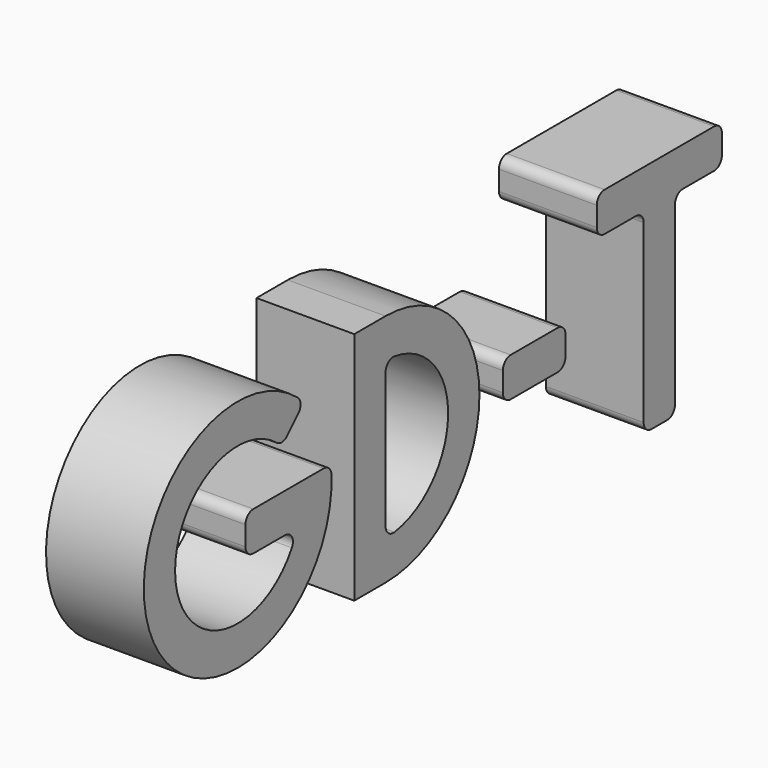
from build123d import *

# Parameters (mm, degrees)
F1_DEPTH = 10
F0_W     = 8
F0_H     = 4
F2_R     = 1
F3_R     = 1
F4_R     = 1
F4_2_R   = 1
F4_3_R   = 1


with BuildPart() as f1:
    # F0 (on Right) → F1 (new body)
    with BuildSketch(Plane.YZ):
        with BuildLine():
            Line((17.6568542495, 17.6568542495), (20.4852813742, 20.4852813742))
            ThreePointArc((20.4852813742, 20.4852813742), (1.2227826555, 6.7225397861), (23.9058808998, 13.5))
            Line((23.9058808998, 13.5), (13, 13.5))
            Line((13, 13.5), (13, 9.5))
            Line((13, 9.5), (19.5993420768, 9.5))
            ThreePointArc((19.5993420768, 9.5), (4.217631911, 10.1466929753), (17.6568542495, 17.6568542495))
        make_face()
    extrude(amount=F1_DEPTH)

    # F3
    f3_edges = [f1.edges().sort_by_distance(p)[0] for p in [
        (5, 19.599342, 9.5),
        (5, 13, 9.5),
        (5, 13, 13.5),
        (5, 23.905881, 13.5),
        (5, 20.485281, 20.485281),
        (5, 17.656854, 17.656854),
    ]]
    fillet(f3_edges, radius=F3_R)


with BuildPart() as f1b:
    # F0 (on Right) → F1, piece 2 (new body)
    with BuildSketch(Plane.YZ):
        with BuildLine():
            Line((26.9058808998, 0), (30.9058808998, 0))
            ThreePointArc((30.9058808998, 0), (42.9058808998, 12), (30.9058808998, 24))
            Line((30.9058808998, 24), (26.9058808998, 24))
            Line((26.9058808998, 24), (26.9058808998, 0))
        make_face()
        with BuildLine():
            ThreePointArc((30.9058808998, 20), (38.9058808998, 12), (30.9058808998, 4))
            Line((30.9058808998, 4), (30.9058808998, 20))
        make_face(mode=Mode.SUBTRACT)
    extrude(amount=F1_DEPTH)

    # F2
    f2_edges = [f1b.edges().sort_by_distance(p)[0] for p in [
        (5, 30.905881, 4),
    ]]
    fillet(f2_edges, radius=F2_R)

    # F4#3
    f4_3_edges = [f1b.edges().sort_by_distance(p)[0] for p in [
        (5, 30.905881, 20),
    ]]
    fillet(f4_3_edges, radius=F4_3_R)


with BuildPart() as f1c:
    # F0 (on Right) → F1, piece 3 (new body)
    with BuildSketch(Plane.YZ):
        with Locations((49.9058808998, 12)):
            Rectangle(F0_W, F0_H)
    extrude(amount=F1_DEPTH)

    # F4
    f4_edges = [f1c.edges().sort_by_distance(p)[0] for p in [
        (5, 53.905881, 14),
        (5, 45.905881, 14),
        (5, 53.905881, 10),
        (5, 45.905881, 10),
    ]]
    fillet(f4_edges, radius=F4_R)


with BuildPart() as f1d:
    # F0 (on Right) → F1, piece 4 (new body)
    with BuildSketch(Plane.YZ):
        Polygon((73.9058808998, 24), (57.9058808998, 24), (57.9058808998, 20), (63.9058808998, 20), (63.9058808998, 0), (67.9058808998, 0), (67.9058808998, 20), (73.9058808998, 20), align=None)
    extrude(amount=F1_DEPTH)

    # F4#2
    f4_2_edges = [f1d.edges().sort_by_distance(p)[0] for p in [
        (5, 67.905881, 20),
        (5, 63.905881, 20),
        (5, 57.905881, 20),
        (5, 57.905881, 24),
        (5, 73.905881, 24),
        (5, 73.905881, 20),
        (5, 67.905881, 0),
        (5, 63.905881, 0),
    ]]
    fillet(f4_2_edges, radius=F4_2_R)


solid = Compound([f1.part, f1b.part, f1c.part, f1d.part])
